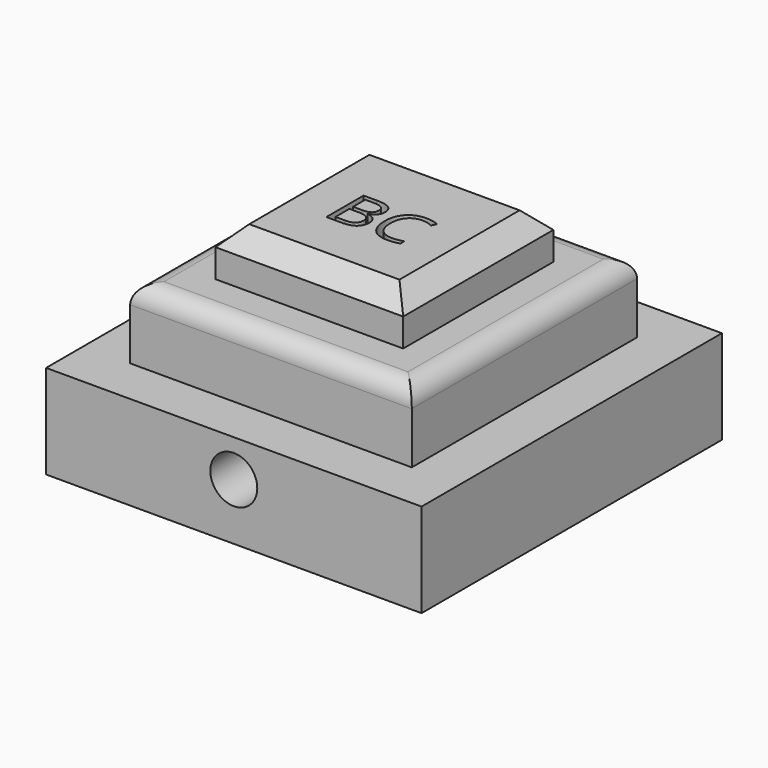
from build123d import *

# Parameters (mm, degrees)
F0_W         = 101.6
F0_H         = 101.6
F1_DEPTH     = 25.4
F3_DEPTH     = 19.05
F5_DEPTH     = 12.7
F6_R         = 6.35
F7_DEPTH     = 121.158
F8_TEXT_SIZE = 17.6388888889
F9_DEPTH     = 25.4
F10_R        = 5.08
F11_SIZE     = 5.08


# Not quite as in the source:
# - Text() gives the source's letters only with a copy of the font that has no kerning and outlines rounded to 1/6400 em; it was checked with that copy


with BuildPart() as f1:
    # F0 (on Top) → F1 (new body)
    with BuildSketch(Plane.XY):
        with Locations((50.8, 50.8)):
            Rectangle(F0_W, F0_H)
    extrude(amount=F1_DEPTH)

    # F2 (on face) → F3 (join)
    with BuildSketch(Plane.XY.offset(25.4)):
        Polygon((12.5850448385, 56.0387484729), (12.5850448385, 12.7164209366), (88.7850448385, 12.7164209366), (88.7850448385, 88.9164209366), (56.0387447476, 88.9164209366), (12.5850448385, 88.9164209366), align=None)
    extrude(amount=F3_DEPTH)

    # F4 (on face) → F5 (join)
    with BuildSketch(Plane.XY.offset(44.45)):
        Polygon((50.6850448385, 76.2711688876), (25.4602152854, 76.2711688876), (25.4602152854, 25.4711688876), (76.2602152854, 25.4711688876), (76.2602152854, 76.2711688876), align=None)
    extrude(amount=F5_DEPTH)

    # F6 (on face) → F7 (cut)
    with BuildSketch(Plane.XZ):
        with Locations((50.7985149404, 15.3080070761)):
            Circle(F6_R)
    extrude(amount=-F7_DEPTH, mode=Mode.SUBTRACT)

    # F8 (on face) → F9 (cut)
    with BuildSketch(Plane.XY.offset(57.15)):
        with Locations((39.4926887709, 43.2670479563)):
            Text('BC', F8_TEXT_SIZE, font='Open Sans', text_align=(TextAlign.LEFT, TextAlign.BOTTOM))
    extrude(amount=-F9_DEPTH, mode=Mode.SUBTRACT)

    # F10
    f10_edges = [f1.edges().sort_by_distance(p)[0] for p in [
        (50.685045, 12.716421, 44.45),
        (12.585045, 50.816421, 44.45),
        (50.685045, 88.916421, 44.45),
        (88.785045, 50.816421, 44.45),
    ]]
    fillet(f10_edges, radius=F10_R)

    # F11
    f11_edges = [f1.edges().sort_by_distance(p)[0] for p in [
        (50.860215, 25.471169, 57.15),
        (76.260215, 50.871169, 57.15),
        (50.860215, 76.271169, 57.15),
        (25.460215, 50.871169, 57.15),
    ]]
    chamfer(f11_edges, length=F11_SIZE)


solid = f1.part
